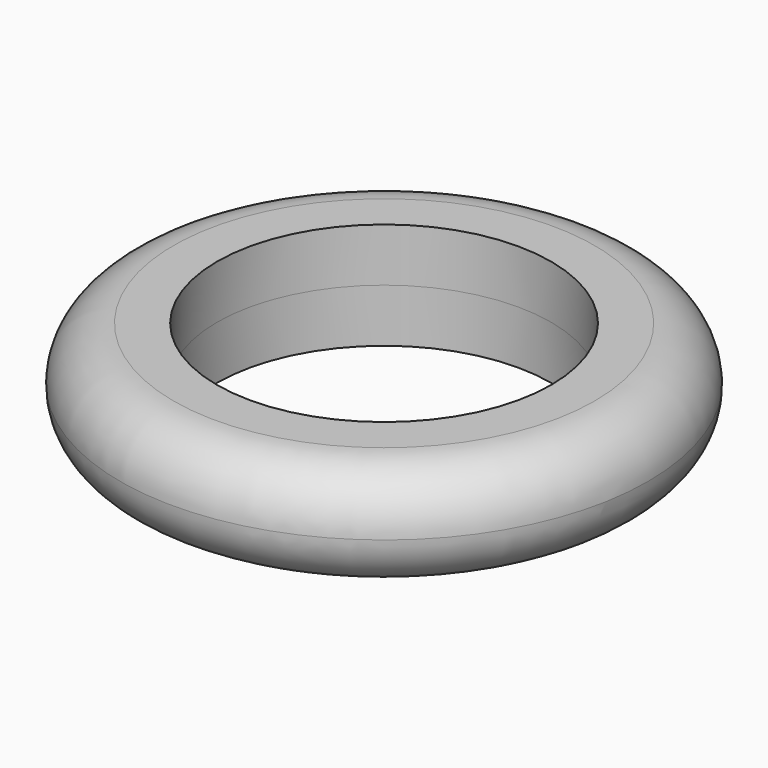
from build123d import *

# Parameters (mm, degrees)
F0_R     = 17.3
F0_R_2   = 10.95
F1_DEPTH = 3.5
F2_DEPTH = 3.5
F3_R     = 3.49999
F4_R     = 3.49999


# Not quite as in the source:
# - a fillet or chamfer is up to 0.001 mm smaller than in the source, because OpenCascade refuses the exact size


with BuildPart() as f1:
    # F0 (on Top) → F1 (new body)
    with BuildSketch(Plane.XY):
        Circle(F0_R)
        Circle(F0_R_2, mode=Mode.SUBTRACT)
    extrude(amount=F1_DEPTH)

    # F2 (add): a face of the model
    f2_faces = [f1.faces().sort_by_distance(p)[0] for p in [
        (-16.8106821074, 0, 0),
    ]]
    extrude(f2_faces, amount=F2_DEPTH)

    # F3 (radius 3.5 in the source; OpenCascade refuses exactly that, so slightly less here)
    f3_edges = [f1.edges().sort_by_distance(p)[0] for p in [
        (-17.3, 0, 3.5),
    ]]
    fillet(f3_edges, radius=F3_R)

    # F4 (radius 3.5 in the source; OpenCascade refuses exactly that, so slightly less here)
    f4_edges = [f1.edges().sort_by_distance(p)[0] for p in [
        (-17.3, 0, -3.5),
    ]]
    fillet(f4_edges, radius=F4_R)


solid = f1.part
